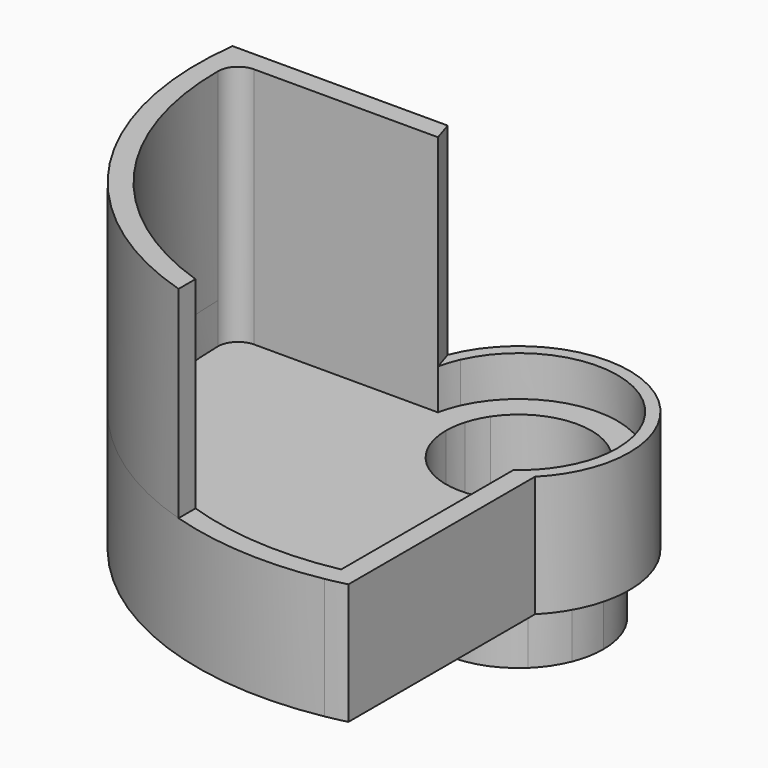
from build123d import *

# Parameters (mm, degrees)
F1_DEPTH    = 2
F2_DEPTH    = 3
F3_DEPTH    = 1.5
F5_DEPTH    = 5
F6_T1_DEPTH = 7.2507051877


# Not quite as in the source:
# - a fillet or chamfer that OpenCascade refuses, or shapes differently, is made with other operations: its cross-section is extruded or revolved along the edge and cut away or added
# - a feature names something its author has since deleted; it is built from what else it names


with BuildPart() as f1:
    # F0 (on Top) → F1 (new body)
    with BuildSketch(Plane.XY):
        with BuildLine():
            ThreePointArc((-2.398436991, 0.5), (-2.3309771289, 0.7543511281), (-2.2366269246, 1))
            Line((-2.2366269246, 1), (-2.556369496, 1))
            ThreePointArc((-2.556369496, 1), (-2.6395896521, 0.7533866658), (-2.6990785465, 0.5))
            Line((-2.6990785465, 0.5), (-2.398436991, 0.5))
        make_face()
        with BuildLine():
            ThreePointArc((-2.2366269246, 1), (0.5112553348, 2.3960630173), (2.45, 0))
            ThreePointArc((2.45, 0), (2.3216373532, -0.7826237921), (1.95, -1.4832396974))
            Line((1.95, -1.4832396974), (1.95, -1.9319743787))
            ThreePointArc((1.95, -1.9319743787), (2.5384813373, -1.0445752725), (2.745, 0))
            ThreePointArc((2.745, 0), (0.5088176164, 2.6974301906), (-2.556369496, 1))
            Line((-2.556369496, 1), (-2.2366269246, 1))
        make_face()
        with BuildLine():
            ThreePointArc((-2.6990785465, 0.5), (-2.6395896521, 0.7533866658), (-2.556369496, 1))
            Line((-2.556369496, 1), (-7.3825808495, 1))
            ThreePointArc((-7.3825808495, 1), (-7.4121089685, 0.7504269711), (-7.43320254, 0.5))
            Line((-7.43320254, 0.5), (-2.6990785465, 0.5))
        make_face()
        with BuildLine():
            ThreePointArc((-2.745, 0), (-2.7334955286, 0.2510521758), (-2.6990785465, 0.5))
            Line((-2.6990785465, 0.5), (-7.43320254, 0.5))
            ThreePointArc((-7.43320254, 0.5), (-7.4457994508, 0.2501410375), (-7.45, 0))
            Line((-7.45, 0), (-2.745, 0))
        make_face()
        with BuildLine():
            Line((1.45, -7.3075303626), (1.45, -2.3307777672))
            ThreePointArc((1.45, -2.3307777672), (-1.3331869711, -2.399507762), (-2.745, 0))
            Line((-2.745, 0), (-7.45, 0))
            ThreePointArc((-7.45, 0), (-4.7275786614, -5.7578207683), (1.45, -7.3075303626))
        make_face()
        with BuildLine():
            Line((1.45, -2.3307777672), (1.45, -1.9748417658))
            ThreePointArc((1.45, -1.9748417658), (-1.1067971811, -2.1857492994), (-2.45, 0))
            Line((-2.45, 0), (-2.745, 0))
            ThreePointArc((-2.745, 0), (-1.3331869711, -2.399507762), (1.45, -2.3307777672))
        make_face()
        with BuildLine():
            Line((1.95, -1.9319743787), (1.95, -1.4832396974))
            ThreePointArc((1.95, -1.4832396974), (1.7176781271, -1.7470208504), (1.45, -1.9748417658))
            Line((1.45, -1.9748417658), (1.45, -2.3307777672))
            ThreePointArc((1.45, -2.3307777672), (1.7116544732, -2.1459878761), (1.95, -1.9319743787))
        make_face()
        with BuildLine():
            ThreePointArc((-2.745, 0), (-2.7334955286, 0.2510521758), (-2.6990785465, 0.5))
            Line((-2.6990785465, 0.5), (-7.43320254, 0.5))
            ThreePointArc((-7.43320254, 0.5), (-7.4457994508, 0.2501410375), (-7.45, 0))
            Line((-7.45, 0), (-2.745, 0))
        make_face()
        with BuildLine():
            Line((1.45, -7.3075303626), (1.45, -2.3307777672))
            ThreePointArc((1.45, -2.3307777672), (-1.3331869711, -2.399507762), (-2.745, 0))
            Line((-2.745, 0), (-7.45, 0))
            ThreePointArc((-7.45, 0), (-4.7275786614, -5.7578207683), (1.45, -7.3075303626))
        make_face()
        with BuildLine():
            Line((1.95, -7.1902712049), (1.95, -1.9319743787))
            ThreePointArc((1.95, -1.9319743787), (1.7116544732, -2.1459878761), (1.45, -2.3307777672))
            Line((1.45, -2.3307777672), (1.45, -7.3075303626))
            ThreePointArc((1.45, -7.3075303626), (1.7010107076, -7.253210501), (1.95, -7.1902712049))
        make_face()
        with BuildLine():
            ThreePointArc((-7.43320254, 0.5), (-7.4121089685, 0.7504269711), (-7.3825808495, 1))
            Line((-7.3825808495, 1), (-7.8868561544, 1))
            ThreePointArc((-7.8868561544, 1), (-7.9145080827, 0.7503744455), (-7.9342611502, 0.5))
            Line((-7.9342611502, 0.5), (-7.43320254, 0.5))
        make_face()
        with BuildLine():
            Line((1.95, -7.7071395472), (1.95, -7.1902712049))
            ThreePointArc((1.95, -7.1902712049), (1.7010107076, -7.253210501), (1.45, -7.3075303626))
            Line((1.45, -7.3075303626), (1.45, -7.8166488983))
            ThreePointArc((1.45, -7.8166488983), (1.700881558, -7.7659192582), (1.95, -7.7071395472))
        make_face()
        with BuildLine():
            ThreePointArc((-2.745, 0), (-2.7334955286, 0.2510521758), (-2.6990785465, 0.5))
            Line((-2.6990785465, 0.5), (-7.43320254, 0.5))
            ThreePointArc((-7.43320254, 0.5), (-7.4457994508, 0.2501410375), (-7.45, 0))
            Line((-7.45, 0), (-2.745, 0))
        make_face()
        with BuildLine():
            Line((1.45, -7.3075303626), (1.45, -2.3307777672))
            ThreePointArc((1.45, -2.3307777672), (-1.3331869711, -2.399507762), (-2.745, 0))
            Line((-2.745, 0), (-7.45, 0))
            ThreePointArc((-7.45, 0), (-4.7275786614, -5.7578207683), (1.45, -7.3075303626))
        make_face()
        with BuildLine():
            Line((1.95, -7.1902712049), (1.95, -1.9319743787))
            ThreePointArc((1.95, -1.9319743787), (1.7116544732, -2.1459878761), (1.45, -2.3307777672))
            Line((1.45, -2.3307777672), (1.45, -7.3075303626))
            ThreePointArc((1.45, -7.3075303626), (1.7010107076, -7.253210501), (1.95, -7.1902712049))
        make_face()
        with BuildLine():
            ThreePointArc((-7.43320254, 0.5), (-7.4121089685, 0.7504269711), (-7.3825808495, 1))
            Line((-7.3825808495, 1), (-7.8868561544, 1))
            ThreePointArc((-7.8868561544, 1), (-7.9145080827, 0.7503744455), (-7.9342611502, 0.5))
            Line((-7.9342611502, 0.5), (-7.43320254, 0.5))
        make_face()
        with BuildLine():
            Line((1.45, -7.8166488983), (1.45, -7.3075303626))
            ThreePointArc((1.45, -7.3075303626), (-4.7275786614, -5.7578207683), (-7.45, 0))
            Line((-7.45, 0), (-7.95, 0))
            ThreePointArc((-7.95, 0), (-5.0830601019, -6.1126917148), (1.45, -7.8166488983))
        make_face()
        with BuildLine():
            Line((1.95, -7.7071395472), (1.95, -7.1902712049))
            ThreePointArc((1.95, -7.1902712049), (1.7010107076, -7.253210501), (1.45, -7.3075303626))
            Line((1.45, -7.3075303626), (1.45, -7.8166488983))
            ThreePointArc((1.45, -7.8166488983), (1.700881558, -7.7659192582), (1.95, -7.7071395472))
        make_face()
        with BuildLine():
            ThreePointArc((-7.45, 0), (-7.4457994508, 0.2501410375), (-7.43320254, 0.5))
            Line((-7.43320254, 0.5), (-7.9342611502, 0.5))
            ThreePointArc((-7.9342611502, 0.5), (-7.9460643134, 0.250123825), (-7.95, 0))
            Line((-7.95, 0), (-7.45, 0))
        make_face()
        with BuildLine():
            ThreePointArc((-2.45, 0), (-2.4370751556, 0.2513258562), (-2.398436991, 0.5))
            Line((-2.398436991, 0.5), (-2.6990785465, 0.5))
            ThreePointArc((-2.6990785465, 0.5), (-2.7334955286, 0.2510521758), (-2.745, 0))
            Line((-2.745, 0), (-2.45, 0))
        make_face()
        with BuildLine():
            ThreePointArc((-2.45, 0), (-1.1067971811, -2.1857492994), (1.45, -1.9748417658))
            Line((1.45, -1.9748417658), (1.45, -1.5190457531))
            ThreePointArc((1.45, -1.5190457531), (-0.8261355821, -1.9306734576), (-2.1, 0))
            Line((-2.1, 0), (-2.45, 0))
        make_face()
        with BuildLine():
            ThreePointArc((-2.1, 0), (-0.8261355821, -1.9306734576), (1.45, -1.5190457531))
            Line((1.45, -1.5190457531), (1.45, -1.0665364504))
            ThreePointArc((1.45, -1.0665364504), (-0.561248608, -1.7102631376), (-1.8, 0))
            Line((-1.8, 0), (-2.1, 0))
        make_face()
        with BuildLine():
            Line((-2.0396078054, 0.5), (-2.398436991, 0.5))
            ThreePointArc((-2.398436991, 0.5), (-2.4370751556, 0.2513258562), (-2.45, 0))
            Line((-2.45, 0), (-2.1, 0))
            ThreePointArc((-2.1, 0), (-2.0848472835, 0.2518170056), (-2.0396078054, 0.5))
        make_face()
        with BuildLine():
            Line((-1.8466185313, 1), (-2.2366269246, 1))
            ThreePointArc((-2.2366269246, 1), (-2.3309771289, 0.7543511281), (-2.398436991, 0.5))
            Line((-2.398436991, 0.5), (-2.0396078054, 0.5))
            ThreePointArc((-2.0396078054, 0.5), (-1.9591295988, 0.7561819986), (-1.8466185313, 1))
        make_face()
        with BuildLine():
            Line((2.1, 0), (2.45, 0))
            ThreePointArc((2.45, 0), (0.5112553348, 2.3960630173), (-2.2366269246, 1))
            Line((-2.2366269246, 1), (-1.8466185313, 1))
            ThreePointArc((-1.8466185313, 1), (0.5158008745, 2.0356692899), (2.1, 0))
        make_face()
        with BuildLine():
            Line((-1.7291616466, 0.5), (-2.0396078054, 0.5))
            ThreePointArc((-2.0396078054, 0.5), (-2.0848472835, 0.2518170056), (-2.1, 0))
            Line((-2.1, 0), (-1.8, 0))
            ThreePointArc((-1.8, 0), (-1.7822024245, 0.2524965704), (-1.7291616466, 0.5))
        make_face()
        with BuildLine():
            Line((-1.4966629547, 1), (-1.8466185313, 1))
            ThreePointArc((-1.8466185313, 1), (-1.9591295988, 0.7561819986), (-2.0396078054, 0.5))
            Line((-2.0396078054, 0.5), (-1.7291616466, 0.5))
            ThreePointArc((-1.7291616466, 0.5), (-1.6321721997, 0.7589558027), (-1.4966629547, 1))
        make_face()
        with BuildLine():
            Line((1.95, 0), (2.1, 0))
            ThreePointArc((2.1, 0), (0.5158008745, 2.0356692899), (-1.8466185313, 1))
            Line((-1.8466185313, 1), (-1.4966629547, 1))
            ThreePointArc((-1.4966629547, 1), (0.522497216, 1.722497216), (1.8, 0))
            Line((1.8, 0), (1.95, 0))
        make_face()
        with BuildLine():
            ThreePointArc((1.45, -1.5190457531), (1.739758749, -1.176112025), (1.95, -0.7794228634))
            Line((1.95, -0.7794228634), (1.95, 0))
            Line((1.95, 0), (1.8, 0))
            ThreePointArc((1.8, 0), (1.7102631376, -0.561248608), (1.45, -1.0665364504))
            Line((1.45, -1.0665364504), (1.45, -1.5190457531))
        make_face()
        with BuildLine():
            ThreePointArc((1.45, -1.9748417658), (1.7176781271, -1.7470208504), (1.95, -1.4832396974))
            Line((1.95, -1.4832396974), (1.95, -0.7794228634))
            ThreePointArc((1.95, -0.7794228634), (1.739758749, -1.176112025), (1.45, -1.5190457531))
            Line((1.45, -1.5190457531), (1.45, -1.9748417658))
        make_face()
        with BuildLine():
            ThreePointArc((1.95, -0.7794228634), (2.0621590627, -0.3968626967), (2.1, 0))
            Line((2.1, 0), (1.95, 0))
            Line((1.95, 0), (1.95, -0.7794228634))
        make_face()
        with BuildLine():
            ThreePointArc((1.95, -1.4832396974), (2.3216373532, -0.7826237921), (2.45, 0))
            Line((2.45, 0), (2.1, 0))
            ThreePointArc((2.1, 0), (2.0621590627, -0.3968626967), (1.95, -0.7794228634))
            Line((1.95, -0.7794228634), (1.95, -1.4832396974))
        make_face()
    extrude(amount=F1_DEPTH)

    # F0 (on Top) → F2 (join)
    with BuildSketch(Plane.XY):
        with BuildLine():
            ThreePointArc((-7.43320254, 0.5), (-7.4121089685, 0.7504269711), (-7.3825808495, 1))
            Line((-7.3825808495, 1), (-7.8868561544, 1))
            ThreePointArc((-7.8868561544, 1), (-7.9145080827, 0.7503744455), (-7.9342611502, 0.5))
            Line((-7.9342611502, 0.5), (-7.43320254, 0.5))
        make_face()
        with BuildLine():
            ThreePointArc((-2.6990785465, 0.5), (-2.6395896521, 0.7533866658), (-2.556369496, 1))
            Line((-2.556369496, 1), (-7.3825808495, 1))
            ThreePointArc((-7.3825808495, 1), (-7.4121089685, 0.7504269711), (-7.43320254, 0.5))
            Line((-7.43320254, 0.5), (-2.6990785465, 0.5))
        make_face()
        with BuildLine():
            ThreePointArc((-2.398436991, 0.5), (-2.3309771289, 0.7543511281), (-2.2366269246, 1))
            Line((-2.2366269246, 1), (-2.556369496, 1))
            ThreePointArc((-2.556369496, 1), (-2.6395896521, 0.7533866658), (-2.6990785465, 0.5))
            Line((-2.6990785465, 0.5), (-2.398436991, 0.5))
        make_face()
        with BuildLine():
            ThreePointArc((-2.2366269246, 1), (0.5112553348, 2.3960630173), (2.45, 0))
            ThreePointArc((2.45, 0), (2.3216373532, -0.7826237921), (1.95, -1.4832396974))
            Line((1.95, -1.4832396974), (1.95, -1.9319743787))
            ThreePointArc((1.95, -1.9319743787), (2.5384813373, -1.0445752725), (2.745, 0))
            ThreePointArc((2.745, 0), (0.5088176164, 2.6974301906), (-2.556369496, 1))
            Line((-2.556369496, 1), (-2.2366269246, 1))
        make_face()
        with BuildLine():
            Line((1.95, -1.9319743787), (1.95, -1.4832396974))
            ThreePointArc((1.95, -1.4832396974), (1.7176781271, -1.7470208504), (1.45, -1.9748417658))
            Line((1.45, -1.9748417658), (1.45, -2.3307777672))
            ThreePointArc((1.45, -2.3307777672), (1.7116544732, -2.1459878761), (1.95, -1.9319743787))
        make_face()
        with BuildLine():
            Line((1.95, -7.1902712049), (1.95, -1.9319743787))
            ThreePointArc((1.95, -1.9319743787), (1.7116544732, -2.1459878761), (1.45, -2.3307777672))
            Line((1.45, -2.3307777672), (1.45, -7.3075303626))
            ThreePointArc((1.45, -7.3075303626), (1.7010107076, -7.253210501), (1.95, -7.1902712049))
        make_face()
        with BuildLine():
            Line((1.95, -7.7071395472), (1.95, -7.1902712049))
            ThreePointArc((1.95, -7.1902712049), (1.7010107076, -7.253210501), (1.45, -7.3075303626))
            Line((1.45, -7.3075303626), (1.45, -7.8166488983))
            ThreePointArc((1.45, -7.8166488983), (1.700881558, -7.7659192582), (1.95, -7.7071395472))
        make_face()
        with BuildLine():
            Line((1.45, -7.8166488983), (1.45, -7.3075303626))
            ThreePointArc((1.45, -7.3075303626), (-4.7275786614, -5.7578207683), (-7.45, 0))
            Line((-7.45, 0), (-7.95, 0))
            ThreePointArc((-7.95, 0), (-5.0830601019, -6.1126917148), (1.45, -7.8166488983))
        make_face()
        with BuildLine():
            ThreePointArc((-7.45, 0), (-7.4457994508, 0.2501410375), (-7.43320254, 0.5))
            Line((-7.43320254, 0.5), (-7.9342611502, 0.5))
            ThreePointArc((-7.9342611502, 0.5), (-7.9460643134, 0.250123825), (-7.95, 0))
            Line((-7.95, 0), (-7.45, 0))
        make_face()
    extrude(amount=F2_DEPTH)

    # F0 (on Top) → F3 (join)
    with BuildSketch(Plane.XY):
        with BuildLine():
            Line((1.95, 0), (2.1, 0))
            ThreePointArc((2.1, 0), (0.5158008745, 2.0356692899), (-1.8466185313, 1))
            Line((-1.8466185313, 1), (-1.4966629547, 1))
            ThreePointArc((-1.4966629547, 1), (0.522497216, 1.722497216), (1.8, 0))
            Line((1.8, 0), (1.95, 0))
        make_face()
        with BuildLine():
            Line((-1.4966629547, 1), (-1.8466185313, 1))
            ThreePointArc((-1.8466185313, 1), (-1.9591295988, 0.7561819986), (-2.0396078054, 0.5))
            Line((-2.0396078054, 0.5), (-1.7291616466, 0.5))
            ThreePointArc((-1.7291616466, 0.5), (-1.6321721997, 0.7589558027), (-1.4966629547, 1))
        make_face()
        with BuildLine():
            Line((-1.7291616466, 0.5), (-2.0396078054, 0.5))
            ThreePointArc((-2.0396078054, 0.5), (-2.0848472835, 0.2518170056), (-2.1, 0))
            Line((-2.1, 0), (-1.8, 0))
            ThreePointArc((-1.8, 0), (-1.7822024245, 0.2524965704), (-1.7291616466, 0.5))
        make_face()
        with BuildLine():
            ThreePointArc((-2.1, 0), (-0.8261355821, -1.9306734576), (1.45, -1.5190457531))
            Line((1.45, -1.5190457531), (1.45, -1.0665364504))
            ThreePointArc((1.45, -1.0665364504), (-0.561248608, -1.7102631376), (-1.8, 0))
            Line((-1.8, 0), (-2.1, 0))
        make_face()
        with BuildLine():
            ThreePointArc((1.45, -1.5190457531), (1.739758749, -1.176112025), (1.95, -0.7794228634))
            Line((1.95, -0.7794228634), (1.95, 0))
            Line((1.95, 0), (1.8, 0))
            ThreePointArc((1.8, 0), (1.7102631376, -0.561248608), (1.45, -1.0665364504))
            Line((1.45, -1.0665364504), (1.45, -1.5190457531))
        make_face()
        with BuildLine():
            ThreePointArc((1.95, -0.7794228634), (2.0621590627, -0.3968626967), (2.1, 0))
            Line((2.1, 0), (1.95, 0))
            Line((1.95, 0), (1.95, -0.7794228634))
        make_face()
    extrude(amount=-F3_DEPTH)

    # F4 (on face) → F5 (join)
    with BuildSketch(Plane.XY.offset(3)):
        with BuildLine():
            Line((-2.398436991, 0.5), (-2.556369496, 1))
            Line((-2.556369496, 1), (-7.8868561544, 1))
            ThreePointArc((-7.8868561544, 1), (-6.6826334673, -4.3063801437), (-2.3478664886, -7.5953948516))
            Line((-2.3478664886, -7.5953948516), (-2.3478664886, -7.0703622928))
            ThreePointArc((-2.3478664886, -7.0703622928), (-6.1842480664, -4.154223857), (-7.43320254, 0.5))
            Line((-7.43320254, 0.5), (-2.398436991, 0.5))
        make_face()
    extrude(amount=F5_DEPTH)

    # F6: fillet of radius 0.5 on 1 edges, made by hand

    # F6_s2 → F6_t1 (join)
    with BuildSketch(Plane.XY.offset(0.7492948123)):
        with BuildLine():
            ThreePointArc((-6.95, 0.5), (-7.3035533906, 0.3535533906), (-7.45, 0))
            ThreePointArc((-7.45, 0), (-7.4457994508, 0.2501410375), (-7.43320254, 0.5))
            Line((-7.43320254, 0.5), (-6.95, 0.5))
        make_face()
    extrude(amount=F6_T1_DEPTH)


solid = f1.part
